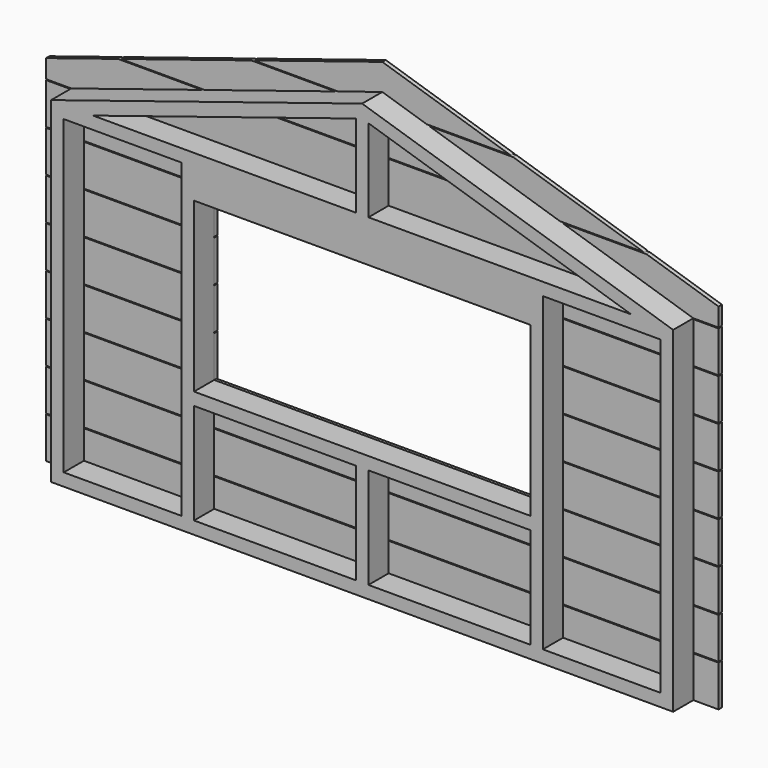
from build123d import *

# Parameters (mm, degrees)
F0_W     = 3.81
F0_H     = 93.98
F0_W_2   = 101.6
F0_H_2   = 3.81
F0_H_3   = 30.48
F0_H_4   = 5.08
F1_DEPTH = 7.62
F2_W     = 203.2
F2_H     = 12.446
F3_DEPTH = 1.27
F0_H_5   = 50.8
F4_DEPTH = 25.4
F6_DEPTH = 2.54


# Not quite as in the source:
# - a feature names something its author has since deleted; it is built from what else it names


with BuildPart() as f1:
    # F0 (on Front) → F1 (new body)
    with BuildSketch(Plane.XZ):
        Polygon((0, 101.6), (0, 97.79), (3.81, 97.79), (39.3699984628, 97.79), (43.18, 97.79), (144.78, 97.79), (148.59, 97.79), (184.15, 97.79), (187.96, 97.79), (187.96, 101.6), (175.2898087158, 101.6), (95.885, 101.6), (92.075, 101.6), (12.6701912842, 101.6), align=None)
        with Locations((1.905, 50.8)):
            Rectangle(F0_W, F0_H)
        Polygon((39.3699984628, 97.79), (39.3699984628, 3.81), (43.18, 3.81), (43.18, 34.29), (43.18, 38.1), (43.18, 88.9), (43.18, 92.71), (43.18, 97.79), align=None)
        with Locations((93.98, 90.805)):
            Rectangle(F0_W_2, F0_H_2)
        Polygon((144.78, 3.81), (148.59, 3.81), (148.59, 97.79), (144.78, 97.79), (144.78, 92.71), (144.78, 88.9), (144.78, 38.1), (144.78, 34.29), align=None)
        with Locations((186.055, 50.8)):
            Rectangle(F0_W, F0_H)
        Polygon((43.18, 38.1), (43.18, 34.29), (92.075, 34.29), (95.885, 34.29), (144.78, 34.29), (144.78, 38.1), align=None)
        with Locations((93.98, 19.05)):
            Rectangle(F0_W, F0_H_3)
        Polygon((0, 3.81), (0, 0), (187.96, 0), (187.96, 3.81), (184.15, 3.81), (148.59, 3.81), (144.78, 3.81), (95.885, 3.81), (92.075, 3.81), (43.18, 3.81), (39.3699984628, 3.81), (3.81, 3.81), align=None)
        Polygon((93.98, 131.2317801788), (0, 101.6), (12.6701912842, 101.6), (92.075, 126.6362400192), (93.98, 127.2368842121), (95.885, 126.6362400192), (175.2898087158, 101.6), (187.96, 101.6), align=None)
        Polygon((92.075, 126.6362400192), (92.075, 101.6), (95.885, 101.6), (95.885, 126.6362400192), (93.98, 127.2368842121), align=None)
        with Locations((93.98, 95.25)):
            Rectangle(F0_W_2, F0_H_4)
    extrude(amount=F1_DEPTH)


with BuildPart() as f3:
    # F2 (on Front) → F3 (new body)
    with BuildSketch(Plane.XZ):
        with Locations((93.98, 6.223)):
            Rectangle(F2_W, F2_H)
    extrude(amount=-F3_DEPTH)


with BuildPart() as f3b:
    # F2 (on Front) → F3, piece 2 (new body)
    with BuildSketch(Plane.XZ):
        with Locations((93.98, 18.923)):
            Rectangle(F2_W, F2_H)
    extrude(amount=-F3_DEPTH)


with BuildPart() as f3c:
    # F2 (on Front) → F3, piece 3 (new body)
    with BuildSketch(Plane.XZ):
        with Locations((93.98, 31.623)):
            Rectangle(F2_W, F2_H)
    extrude(amount=-F3_DEPTH)


with BuildPart() as f3d:
    # F2 (on Front) → F3, piece 4 (new body)
    with BuildSketch(Plane.XZ):
        with Locations((93.98, 44.323)):
            Rectangle(F2_W, F2_H)
    extrude(amount=-F3_DEPTH)


with BuildPart() as f3e:
    # F2 (on Front) → F3, piece 5 (new body)
    with BuildSketch(Plane.XZ):
        with Locations((93.98, 57.023)):
            Rectangle(F2_W, F2_H)
    extrude(amount=-F3_DEPTH)


with BuildPart() as f3f:
    # F2 (on Front) → F3, piece 6 (new body)
    with BuildSketch(Plane.XZ):
        with Locations((93.98, 69.723)):
            Rectangle(F2_W, F2_H)
    extrude(amount=-F3_DEPTH)


with BuildPart() as f3g:
    # F2 (on Front) → F3, piece 7 (new body)
    with BuildSketch(Plane.XZ):
        with Locations((93.98, 82.423)):
            Rectangle(F2_W, F2_H)
    extrude(amount=-F3_DEPTH)


with BuildPart() as f3h:
    # F2 (on Front) → F3, piece 8 (new body)
    with BuildSketch(Plane.XZ):
        with Locations((93.98, 95.123)):
            Rectangle(F2_W, F2_H)
    extrude(amount=-F3_DEPTH)


with BuildPart() as f3i:
    # F2 (on Front) → F3, piece 9 (new body)
    with BuildSketch(Plane.XZ):
        with Locations((93.98, 107.823)):
            Rectangle(F2_W, F2_H)
    extrude(amount=-F3_DEPTH)


with BuildPart() as f3j:
    # F2 (on Front) → F3, piece 10 (new body)
    with BuildSketch(Plane.XZ):
        with Locations((93.98, 120.523)):
            Rectangle(F2_W, F2_H)
    extrude(amount=-F3_DEPTH)


with BuildPart() as f3k:
    # F2 (on Front) → F3, piece 11 (new body)
    with BuildSketch(Plane.XZ):
        with Locations((93.98, 133.223)):
            Rectangle(F2_W, F2_H)
    extrude(amount=-F3_DEPTH)


with BuildPart() as f4_tool:
    # F0 (on Front) → F4 (new body)
    with BuildSketch(Plane.XZ):
        with Locations((93.98, 63.5)):
            Rectangle(F0_W_2, F0_H_5)
    extrude(amount=-F4_DEPTH)


with BuildPart() as f3d_1:
    add(f3d.part)

    # F4: cut by f4_tool
    add(f4_tool.part, mode=Mode.SUBTRACT)


with BuildPart() as f3e_1:
    add(f3e.part)

    # F4: cut by f4_tool
    add(f4_tool.part, mode=Mode.SUBTRACT)


with BuildPart() as f3f_1:
    add(f3f.part)

    # F4: cut by f4_tool
    add(f4_tool.part, mode=Mode.SUBTRACT)


with BuildPart() as f3g_1:
    add(f3g.part)

    # F4: cut by f4_tool
    add(f4_tool.part, mode=Mode.SUBTRACT)


with BuildPart() as f6_tool:
    # F5 (on Front) → F6 (new body)
    with BuildSketch(Plane.XZ):
        Polygon((-10.16, 141.605), (-10.16, 106.3863562386), (93.98, 139.2215721124), (198.12, 106.3863562386), (198.12, 141.605), align=None)
    extrude(amount=-F6_DEPTH)


with BuildPart() as f3i_1:
    add(f3i.part)

    # F6: cut by f6_tool
    add(f6_tool.part, mode=Mode.SUBTRACT)


with BuildPart() as f3j_1:
    add(f3j.part)

    # F6: cut by f6_tool
    add(f6_tool.part, mode=Mode.SUBTRACT)


with BuildPart() as f3k_1:
    add(f3k.part)

    # F6: cut by f6_tool
    add(f6_tool.part, mode=Mode.SUBTRACT)


solid = Compound([f1.part, f3.part, f3b.part, f3c.part, f3h.part, f3d_1.part, f3e_1.part, f3f_1.part, f3g_1.part, f3i_1.part, f3j_1.part, f3k_1.part])
